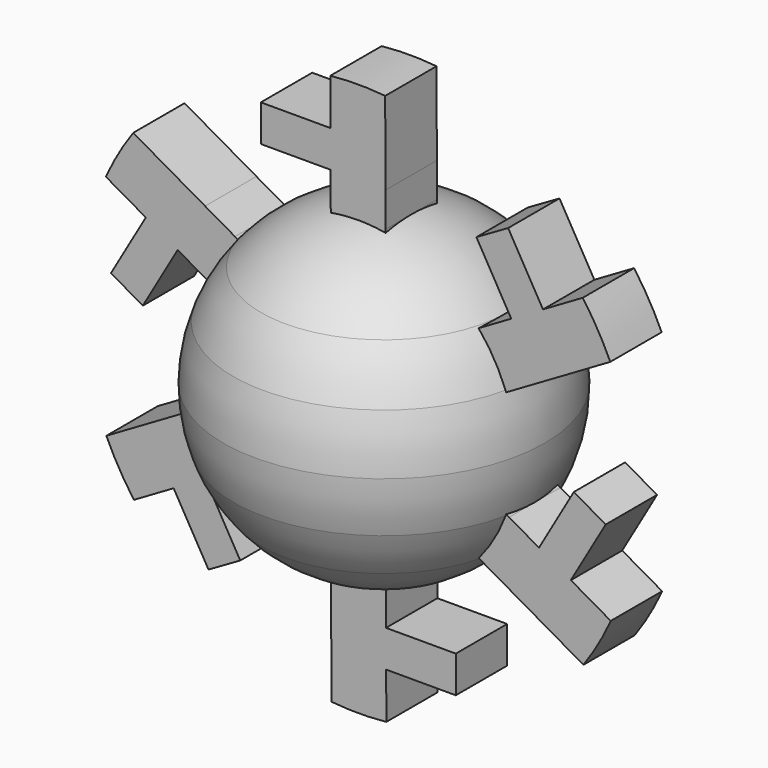
from build123d import *

# Parameters (mm, degrees)
F4_DEPTH = 6.35


# Not quite as in the source:
# - the program builds the solid bodies; features that only make, move or delete a surface that nothing else refers to are left out


with BuildPart() as f2:
    # F0 (on Front) → F2 (revolve)
    with BuildSketch(Plane.XZ):
        with BuildLine():
            ThreePointArc((24.3612137616, 20.3615756773), (15.8531486732, 27.508910868), (5.403325821, 31.2868434022))
            ThreePointArc((5.403325821, 31.2868434022), (2.7115698388, 31.6339989412), (0, 31.75))
            Line((0, 31.75), (0, -31.75))
            ThreePointArc((0, -31.75), (2.736702771, -31.6318345649), (5.4530349168, -31.2782178232))
            ThreePointArc((5.4530349168, -31.2782178232), (15.8968413055, -27.483684915), (24.39353828, -20.322839127))
            ThreePointArc((24.39353828, -20.322839127), (27.508910868, -15.8531486732), (29.8142486784, -10.9166421459))
            ThreePointArc((29.8142486784, -10.9166421459), (31.2623167371, -5.5434693316), (31.75, 0))
            ThreePointArc((31.75, 0), (31.2579024825, 5.5683060617), (29.796864101, 10.9640042752))
            ThreePointArc((29.796864101, 10.9640042752), (27.483684915, 15.8968413055), (24.3612137616, 20.3615756773))
        make_face()
    revolve(axis=Axis((0, 0, 0), (0, 0, -1)))

    # F3 (on Front) → F4 (join, symmetric)
    with BuildSketch(Plane.XZ):
        with BuildLine():
            Line((5.376374884, 38.1001170391), (5.3115624093, 54.484895228))
            ThreePointArc((5.3115624093, 54.484895228), (-0.1171664817, 54.7430614347), (-5.5447405359, 54.4616595011))
            Line((-5.5447405359, 54.4616595011), (-5.5087377694, 45.3600575994))
            Line((-5.5087377694, 45.3600575994), (-19.2836534145, 45.3600575994))
            Line((-19.2836534145, 45.3600575994), (-19.2836534145, 38.1001170391))
            Line((-19.2836534145, 38.1001170391), (-5.4800199737, 38.1001170391))
            Line((-5.4800199737, 38.1001170391), (-5.4530349168, 31.2782178232))
            Line((-5.4530349168, 31.2782178232), (-5.4530349168, 22.3882178232))
            Line((-5.4530349168, 22.3882178232), (5.403325821, 22.3882178232))
            Line((5.403325821, 22.3882178232), (5.403325821, 31.2868434022))
            Line((5.403325821, 31.2868434022), (5.376374884, 38.1001170391))
        make_face()
        with BuildLine():
            Line((22.0904282909, 6.5146914857), (29.796864101, 10.9640042752))
            Line((29.796864101, 10.9640042752), (49.8410845946, 22.6424996338))
            ThreePointArc((49.8410845946, 22.6424996338), (47.3502986425, 27.472999867), (44.3928103923, 32.0327159121))
            Line((44.3928103923, 32.0327159121), (36.5285933135, 27.4507356508))
            Line((36.5285933135, 27.4507356508), (29.6411354909, 39.3801625345))
            Line((29.6411354909, 39.3801625345), (23.3538425357, 35.7501922543))
            Line((23.3538425357, 35.7501922543), (30.2556592562, 23.79589503))
            Line((30.2556592562, 23.79589503), (24.3612137616, 20.3615756773))
            Line((24.3612137616, 20.3615756773), (16.6622479219, 15.9165756773))
            Line((16.6622479219, 15.9165756773), (22.0904282909, 6.5146914857))
        make_face()
        with BuildLine():
            Line((16.6871024699, -15.8735263375), (24.39353828, -20.322839127))
            Line((24.39353828, -20.322839127), (30.307481801, -23.7061357493))
            Line((30.307481801, -23.7061357493), (44.5295221853, -31.8423955942))
            ThreePointArc((44.5295221853, -31.8423955942), (47.4674651242, -27.2700615677), (49.9375509282, -22.4289435891))
            Line((49.9375509282, -22.4289435891), (42.0373310829, -17.9093219486))
            Line((42.0373310829, -17.9093219486), (48.9247889055, -5.9798950649))
            Line((48.9247889055, -5.9798950649), (42.6374959503, -2.3499247848))
            Line((42.6374959503, -2.3499247848), (35.7356792298, -14.3042220091))
            Line((35.7356792298, -14.3042220091), (29.8142486784, -10.9166421459))
            Line((29.8142486784, -10.9166421459), (22.1152828388, -6.4716421459))
            Line((22.1152828388, -6.4716421459), (16.6871024699, -15.8735263375))
        make_face()
        with BuildLine():
            Line((-5.403325821, -22.3882178232), (-5.403325821, -31.2868434022))
            Line((-5.403325821, -31.2868434022), (-5.3115624093, -54.484895228))
            ThreePointArc((-5.3115624093, -54.484895228), (0.1171664817, -54.7430614347), (5.5447405359, -54.4616595011))
            Line((5.5447405359, -54.4616595011), (5.5087377694, -45.3600575994))
            Line((5.5087377694, -45.3600575994), (19.2836534145, -45.3600575994))
            Line((19.2836534145, -45.3600575994), (19.2836534145, -38.1001170391))
            Line((19.2836534145, -38.1001170391), (5.4800199737, -38.1001170391))
            Line((5.4800199737, -38.1001170391), (5.4530349168, -31.2782178232))
            Line((5.4530349168, -31.2782178232), (5.4530349168, -22.3882178232))
            Line((5.4530349168, -22.3882178232), (-5.403325821, -22.3882178232))
        make_face()
        with BuildLine():
            Line((-29.796864101, -10.9640042752), (-49.8410845946, -22.6424996338))
            ThreePointArc((-49.8410845946, -22.6424996338), (-47.3502986425, -27.472999867), (-44.3928103923, -32.0327159121))
            Line((-44.3928103923, -32.0327159121), (-36.5285933135, -27.4507356508))
            Line((-36.5285933135, -27.4507356508), (-29.6411354909, -39.3801625345))
            Line((-29.6411354909, -39.3801625345), (-23.3538425357, -35.7501922543))
            Line((-23.3538425357, -35.7501922543), (-30.2556592562, -23.79589503))
            Line((-30.2556592562, -23.79589503), (-24.3612137616, -20.3615756773))
            Line((-24.3612137616, -20.3615756773), (-16.6622479219, -15.9165756773))
            Line((-16.6622479219, -15.9165756773), (-22.0904282909, -6.5146914857))
            Line((-22.0904282909, -6.5146914857), (-29.796864101, -10.9640042752))
        make_face()
        with BuildLine():
            Line((-16.6871024699, 15.8735263375), (-24.39353828, 20.322839127))
            Line((-24.39353828, 20.322839127), (-30.307481801, 23.7061357493))
            Line((-30.307481801, 23.7061357493), (-44.5295221853, 31.8423955942))
            ThreePointArc((-44.5295221853, 31.8423955942), (-47.4674651242, 27.2700615677), (-49.9375509282, 22.4289435891))
            Line((-49.9375509282, 22.4289435891), (-42.0373310829, 17.9093219486))
            Line((-42.0373310829, 17.9093219486), (-48.9247889055, 5.9798950649))
            Line((-48.9247889055, 5.9798950649), (-42.6374959503, 2.3499247848))
            Line((-42.6374959503, 2.3499247848), (-35.7356792298, 14.3042220091))
            Line((-35.7356792298, 14.3042220091), (-29.8142486784, 10.9166421459))
            Line((-29.8142486784, 10.9166421459), (-22.1152828388, 6.4716421459))
            Line((-22.1152828388, 6.4716421459), (-16.6871024699, 15.8735263375))
        make_face()
    extrude(amount=F4_DEPTH, both=True)


solid = f2.part
